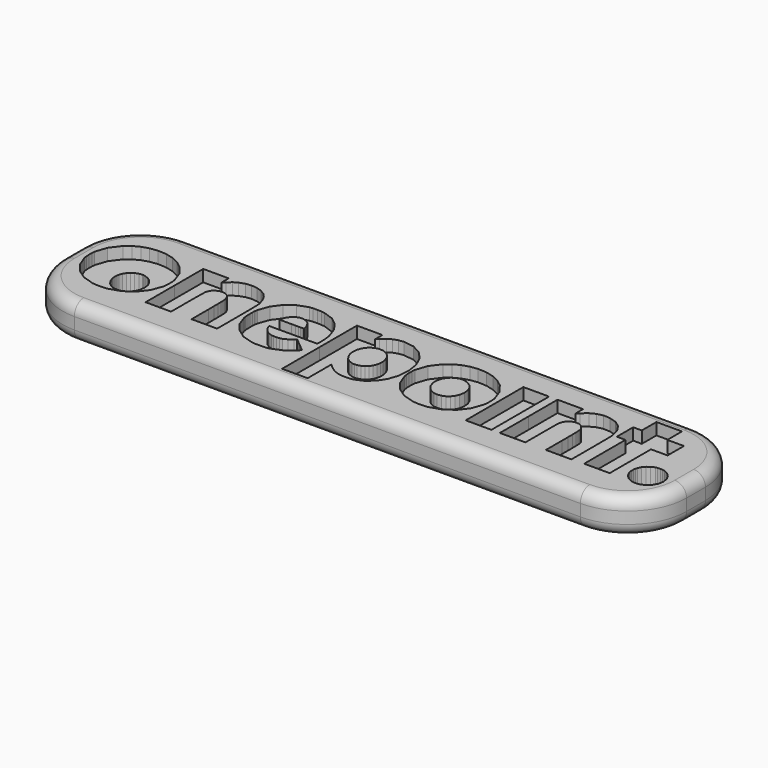
from build123d import *

# Parameters (mm, degrees)
F0_W     = 52.8722088784
F0_H     = 12
F1_DEPTH = 3
F2_DEPTH = 1
F3_R     = 5
F4_DEPTH = 3
F5_R     = 1
F6_R     = 1


# Not quite as in the source:
# - a feature names something its author has since deleted; it is built from what else it names


with BuildPart() as f1:
    # F0 (on Top) → F1 (new body)
    with BuildSketch(Plane.XY):
        with Locations((0.0200578943, 0)):
            Rectangle(F0_W, F0_H)
        Polygon((-4.8085591433, -0.7883964354), (-4.8082865964, -0.7883964354), (-4.8082865964, 3.167022304), (-2.6444276898, 3.167022304), (-2.6444276898, 2.3789256702), (-2.4436151294, 2.5936381229), (-2.0997154432, 2.8928946258), (-1.743660165, 3.1061898346), (-1.3576792365, 3.2388656685), (-0.9247112214, 3.2959369906), (-0.0383886827, 3.1815763088), (0.7376068685, 2.7766806251), (1.3524181794, 2.1192429781), (1.7551879973, 1.2465477846), (1.9036170423, 0.2741549329), (1.8268133242, -0.730998057), (1.5597173562, -1.5324494892), (1.1208078185, -2.1981180527), (0.5367943081, -2.6997133788), (-0.1652865222, -3.0096537204), (-0.3063568008, -3.0427409148), (-0.4323279808, -3.0595843136), (-0.5826103448, -3.0657983831), (-0.7957965348, -3.0669430801), (-1.017595207, -3.0657983831), (-1.170439512, -3.0595843136), (-1.2937942417, -3.0427409148), (-1.4262520381, -3.0096537204), (-1.7128078552, -2.9111552686), (-1.9763607135, -2.7819135257), (-2.2265042639, -2.6124983688), (-2.4725596108, -2.3933161469), (-2.6444276898, -2.2356750164), (-2.6444276898, -4.7579331046), (-4.8085591433, -4.7579331046), align=None, mode=Mode.SUBTRACT)
        Polygon((23.3377414195, -2.9093019496), (23.3371963256, -2.9093019496), (23.0014730467, -2.7620721109), (22.7173156423, -2.5293715624), (22.5026031897, -2.2318048503), (22.3769045565, -1.8917208208), (22.3636042675, -1.7213790045), (22.3680740368, -1.5297785295), (22.391131505, -1.3434654644), (22.4352295945, -1.1894219531), (22.5715030475, -0.9104974493), (22.7643027289, -0.6771427883), (23.010957679, -0.492083439), (23.3091239943, -0.3583719269), (23.4737423256, -0.3258298263), (23.6813685587, -0.315200497), (23.8893218481, -0.3258298263), (24.0542672357, -0.3583719269), (24.4497327965, -0.5594570342), (24.7475175462, -0.8507551675), (24.9347027613, -1.2148233247), (25.000005, -1.6338914476), (24.9261447884, -2.0606453933), (24.722334212, -2.4379593301), (24.4135930767, -2.7319284231), (24.0255953012, -2.9093019496), (23.8674635862, -2.9333405867), (23.6757540924, -2.9412989564), (23.487097124, -2.9333405867), align=None, mode=Mode.SUBTRACT)
        Polygon((-22.2201146743, -3.0240987065), (-22.2201146743, -3.0237716502), (-23.191886119, -2.7287123696), (-23.9953925549, -2.1889604767), (-24.5921830643, -1.4398380504), (-24.9429182269, -0.515958548), (-24.9837294006, -0.2705573137), (-24.999995, 0.0270093984), (-24.9952635857, 0.3327525177), (-24.9713067127, 0.6018108234), (-24.6489600358, 1.5727864313), (-24.0252582449, 2.3931526187), (-23.5512010582, 2.774663778), (-23.0150413335, 3.0576219759), (-22.4253479455, 3.2415911376), (-21.7898230698, 3.3246634346), (-21.0584761528, 3.2880331304), (-20.3765147352, 3.1170917108), (-19.7563669559, 2.8169085484), (-19.2101502503, 2.3931526187), (-18.6118825367, 1.6049469662), (-18.2930844206, 0.6879356458), (-18.2635130813, 0.4265086534), (-18.2575933625, 0.1219102311), (-18.2732702605, -0.1827427006), (-18.3078673648, -0.4444422398), (-18.6444137354, -1.3751354149), (-19.2358786783, -2.1404471274), (-20.0370139561, -2.6990592662), (-21.001993532, -3.0096537204), (-21.6168157447, -3.0542423943), align=None, mode=Mode.SUBTRACT)
        Polygon((-17.8210931395, 0.1002700068), (-17.8205044381, 0.1002700068), (-17.8205044381, 3.152577318), (-15.6566346297, 3.152577318), (-15.6566346297, 2.3644806842), (-15.4274226816, 2.5936381229), (-15.1086518202, 2.8857538969), (-14.7682407344, 3.0810065005), (-14.3237712399, 3.2424632877), (-13.8331322994, 3.2977903096), (-13.3374784959, 3.2484048102), (-12.8764381495, 3.0951789396), (-12.4913838805, 2.8550651153), (-12.1906556243, 2.5365122914), (-11.9676577457, 2.1322707202), (-11.8159036283, 1.6336734101), (-11.8017311892, 1.5656457023), (-11.7907748036, 1.467801363), (-11.7828164339, 1.3219887682), (-11.7766023645, 1.1104923691), (-11.7718600483, 0.8162507292), (-11.7680443916, 0.4205671309), (-11.7642287349, -0.0940014279), (-11.7594319094, -0.7451704961), (-11.7594319094, -2.952255342), (-13.9233453254, -2.952255342), (-13.9233453254, -1.1751950046), (-13.9283601884, -0.5916720785), (-13.9327754483, -0.1492739405), (-13.9369181613, 0.1739121808), (-13.9416604775, 0.3996355285), (-13.9482016032, 0.5492092706), (-13.9561599729, 0.6447642159), (-13.9671163585, 0.7077770606), (-13.9812887976, 0.759451954), (-14.0975027984, 1.0067065072), (-14.2539447225, 1.1894764625), (-14.4530129828, 1.3078163291), (-14.6978691232, 1.3613445415), (-14.9862237499, 1.3444466333), (-15.2408370696, 1.2358639459), (-15.4496079997, 1.0472069775), (-15.6007625139, 0.7881238885), (-15.6152074999, 0.7408097456), (-15.6261638855, 0.68139452), (-15.6341767646, 0.5879654406), (-15.6403363247, 0.4389367923), (-15.6450786408, 0.2127228602), (-15.6489488069, -0.1125891269), (-15.6527644636, -0.5583123372), (-15.6572342328, -1.1464685607), (-15.6572342328, -2.952255342), (-17.8210931395, -2.952255342), align=None, mode=Mode.SUBTRACT)
        Polygon((-8.6758907227, -3.0524980941), (-8.6776350229, -3.0524980941), (-9.6970149612, -2.7478996718), (-10.5120937387, -2.1641587082), (-11.0334759702, -1.472380151), (-11.3285897601, -0.6307553049), (-11.3557899414, -0.4902301201), (-11.3732329434, -0.3474700506), (-11.3827175757, -0.1670439988), (-11.3853885354, 0.0858250207), (-11.3823905194, 0.3451806566), (-11.3726333402, 0.5250071053), (-11.3552448476, 0.6646056306), (-11.3285897601, 0.8024053464), (-11.0118357458, 1.6928705981), (-10.4689223088, 2.4218245533), (-9.7632438594, 2.9555804143), (-8.9068469709, 3.253092617), (-8.6205091914, 3.2850351144), (-8.2600931627, 3.2942471998), (-7.8972242118, 3.2791481012), (-7.6026555157, 3.238647631), (-6.7645737793, 2.9502930043), (-6.0979785563, 2.4363240487), (-5.6126815352, 1.7324444089), (-5.3098274131, 0.8455222669), (-5.2702536023, 0.5696502885), (-5.2400554051, 0.2384512882), (-5.2234845532, -0.0792293856), (-5.2234845532, -0.315200497), (-5.2518294315, -0.501513562), (-9.3075999417, -0.501513562), (-9.2924463338, -0.5589119404), (-9.2655732088, -0.6446006877), (-9.2061034739, -0.7738424306), (-9.0623622356, -1.0037084912), (-8.8713613638, -1.1947093631), (-8.6400780592, -1.3399223547), (-8.3751079571, -1.4330243778), (-8.1636115579, -1.4606061247), (-7.9184828705, -1.4600065215), (-7.6760251428, -1.4351502437), (-7.4722690758, -1.3901800041), (-7.1499005952, -1.2269789168), (-6.8272595677, -0.9888819395), (-6.6553914887, -0.8454677575), (-6.0532808637, -1.3470085742), (-5.4514972949, -1.8486039003), (-5.5662395424, -1.9778456432), (-6.3348218177, -2.6278700143), (-7.2859560107, -3.0096537204), (-7.4329133025, -3.0365268454), (-7.5798705943, -3.0540243568), (-7.7697267691, -3.063781536), (-8.04538071, -3.0667250426), (-8.2488097208, -3.0723395088), (-8.4360494453, -3.070213643), (-8.5857322061, -3.0625823296), align=None, mode=Mode.SUBTRACT)
        Polygon((5.5113204389, -3.0542423943), (4.9080106075, -3.0237716502), (3.936217359, -2.7287123696), (3.1327490797, -2.1889604767), (2.5359258646, -1.4398380504), (2.1852125058, -0.515958548), (2.1443849792, -0.2705573137), (2.1278141273, 0.0270093984), (2.1328834998, 0.3327525177), (2.1568131181, 0.6018108234), (2.4791815987, 1.5727864313), (3.1028234294, 2.3931526187), (3.5769460273, 2.774663778), (4.113100301, 3.0576219759), (4.7027827872, 3.2415911376), (5.3382531535, 3.3246634346), (6.0696600308, 3.2880331304), (6.75157239, 3.1170917108), (7.3714530733, 2.8169085484), (7.9176915826, 2.3931526187), (8.5159320416, 1.6049469662), (8.8350299593, 0.6879356458), (8.8646285533, 0.4265086534), (8.8705700759, 0.1219102311), (8.8548713741, -0.1827427006), (8.820257917, -0.4444422398), (8.4836624879, -1.3751354149), (7.8919631547, -2.1404471274), (7.0908387788, -2.6990592662), (6.1258592029, -3.0096537204), align=None, mode=Mode.SUBTRACT)
        Polygon((9.2931267991, -2.9377013372), (9.2931267991, 0.1144969553), (9.2931267991, 3.167022304), (11.4714852012, 3.167022304), (11.4714852012, -2.9377013372), align=None, mode=Mode.SUBTRACT)
        Polygon((12.186811811, 0.1144969553), (12.1880655268, 0.1144969553), (12.1880655268, 3.167022304), (14.3519244334, 3.167022304), (14.3519244334, 2.3501992263), (14.5810818721, 2.5794656838), (15.0143769435, 2.9532365109), (15.4801050967, 3.1940044477), (15.9837717792, 3.3030777196), (16.530228326, 3.2814920046), (17.1752923435, 3.08809272), (17.6818480232, 2.7119779895), (18.0352323417, 2.16928259), (18.221000313, 1.4760322796), (18.2316296423, 1.248891688), (18.2404601621, 0.754164544), (18.2470012878, 0.0473413976), (18.2493451912, -0.8170683699), (18.2493451912, -2.9377013372), (16.0852137377, -2.9377013372), (16.0852137377, -1.2038669391), (16.0849411908, -0.5769545456), (16.0831423812, -0.0996158942), (16.0781275181, 0.2516970678), (16.0689699421, 0.5016225808), (16.0535982966, 0.6734361504), (16.0304863189, 0.7913944514), (15.9982712746, 0.878991027), (15.9556994479, 0.9599919675), (15.7593021473, 1.2034308641), (15.4917155949, 1.347117593), (15.1837921003, 1.3835298596), (14.8668200485, 1.303946163), (14.6334653874, 1.1356757032), (14.4651949276, 0.9026480984), (14.4273109076, 0.8157056354), (14.39891152, 0.7224945935), (14.3785795208, 0.6000665232), (14.3649521755, 0.4265086534), (14.3566667496, 0.1787090064), (14.3525240366, -0.1652451892), (14.350725227, -0.6280843452), (14.350725227, -1.2325388736), (14.350725227, -2.9377013372), (12.186811811, -2.9377013372), align=None, mode=Mode.SUBTRACT)
        Polygon((19.2957072732, -2.8948569636), (19.2957072732, -0.7165530709), (19.2957072732, 1.4760322796), (18.5648999991, 1.4760322796), (18.5648999991, 3.2099756964), (19.2957072732, 3.2099756964), (19.2957072732, 4.7579331046), (21.4595661799, 4.7579331046), (21.4595661799, 3.2099756964), (22.8643274435, 3.2099756964), (22.8643274435, 1.4760322796), (21.4595661799, 1.4760322796), (21.4595661799, -2.8948569636), align=None, mode=Mode.SUBTRACT)
        Polygon((-4.8082865964, 3.167022304), (-4.8082865964, -0.7883964354), (-4.8085591433, -0.7883964354), (-4.8085591433, -4.7579331046), (-2.6444276898, -4.7579331046), (-2.6444276898, -2.2356750164), (-2.4725596108, -2.3933161469), (-2.2265042639, -2.6124983688), (-1.9763607135, -2.7819135257), (-1.7128078552, -2.9111552686), (-1.4262520381, -3.0096537204), (-1.2937942417, -3.0427409148), (-1.170439512, -3.0595843136), (-1.017595207, -3.0657983831), (-0.7957965348, -3.0669430801), (-0.5826103448, -3.0657983831), (-0.4323279808, -3.0595843136), (-0.3063568008, -3.0427409148), (-0.1652865222, -3.0096537204), (0.5367943081, -2.6997133788), (1.1208078185, -2.1981180527), (1.5597173562, -1.5324494892), (1.8268133242, -0.730998057), (1.9036170423, 0.2741549329), (1.7551879973, 1.2465477846), (1.3524181794, 2.1192429781), (0.7376068685, 2.7766806251), (-0.0383886827, 3.1815763088), (-0.9247112214, 3.2959369906), (-1.3576792365, 3.2388656685), (-1.743660165, 3.1061898346), (-2.0997154432, 2.8928946258), (-2.4436151294, 2.5936381229), (-2.6444276898, 2.3789256702), (-2.6444276898, 3.167022304), align=None)
        Polygon((-1.0051670681, -1.1766667579), (-1.2541659216, -1.2467658221), (-1.481851607, -1.2680789902), (-1.6986899255, -1.2467658221), (-2.0156619773, -1.1225389423), (-2.2880453553, -0.9098978461), (-2.498615095, -0.6219247851), (-2.6299281944, -0.2723016139), (-2.6618161824, -0.0986892347), (-2.6725000211, 0.1148240116), (-2.6618161824, 0.3282827484), (-2.6299281944, 0.5016225808), (-2.4852602966, 0.8614935156), (-2.2576291206, 1.1554626086), (-1.9650772716, 1.3660323483), (-1.626846561, 1.4760322796), (-1.1787794473, 1.4530293207), (-0.7815695863, 1.2702593654), (-0.4701574914, 0.9502347883), (-0.2797562227, 0.5158495293), (-0.2312428735, 0.2260231493), (-0.2351130395, -0.0733423724), (-0.2900584958, -0.3648585432), (-0.3944439608, -0.6307553049), (-0.5553556542, -0.8536986741), (-0.7653257907, -1.0406658517), align=None, mode=Mode.SUBTRACT)
        Polygon((-23.191886119, -2.7287123696), (-22.2201146743, -3.0237716502), (-22.2201146743, -3.0240987065), (-21.6168157447, -3.0542423943), (-21.001993532, -3.0096537204), (-20.0370139561, -2.6990592662), (-19.2358786783, -2.1404471274), (-18.6444137354, -1.3751354149), (-18.3078673648, -0.4444422398), (-18.2732702605, -0.1827427006), (-18.2575933625, 0.1219102311), (-18.2635130813, 0.4265086534), (-18.2930844206, 0.6879356458), (-18.6118825367, 1.6049469662), (-19.2101502503, 2.3931526187), (-19.7563669559, 2.8169085484), (-20.3765147352, 3.1170917108), (-21.0584761528, 3.2880331304), (-21.7898230698, 3.3246634346), (-22.4253479455, 3.2415911376), (-23.0150413335, 3.0576219759), (-23.5512010582, 2.774663778), (-24.0252582449, 2.3931526187), (-24.6489600358, 1.5727864313), (-24.9713067127, 0.6018108234), (-24.9952635857, 0.3327525177), (-24.999995, 0.0270093984), (-24.9837294006, -0.2705573137), (-24.9429182269, -0.515958548), (-24.5921830643, -1.4398380504), (-23.9953925549, -2.1889604767), align=None)
        Polygon((-21.0155936226, -1.0734259898), (-21.3030488445, -1.1894219531), (-21.3033431951, -1.1894219531), (-21.6239183171, -1.221582488), (-21.9338423059, -1.1894219531), (-22.24850316, -1.0551108377), (-22.5161387709, -0.8365827284), (-22.7216772947, -0.5505720051), (-22.8509081357, -0.2149577449), (-22.8837336851, -0.0564444643), (-22.8943793672, 0.1399528363), (-22.8837336851, 0.3413104906), (-22.8509081357, 0.5158495293), (-22.7624830175, 0.7710624522), (-22.614615419, 1.0085598262), (-22.4238707413, 1.2110621774), (-22.2059204314, 1.3613445415), (-21.9214250689, 1.4600610309), (-21.6472810379, 1.5047042141), (-21.5417018174, 1.4941293942), (-21.4035968491, 1.4615872936), (-21.0717818927, 1.3424297862), (-20.7911348925, 1.1410176226), (-20.5693362203, 0.8674350382), (-20.4146658511, 0.5302945153), (-20.364986001, 0.091439487), (-20.4430543368, -0.3583719269), (-20.5855963688, -0.6594272394), (-20.7763464974, -0.8974697072), align=None, mode=Mode.SUBTRACT)
        Polygon((3.936217359, -2.7287123696), (4.9080106075, -3.0237716502), (5.5113204389, -3.0542423943), (6.1258592029, -3.0096537204), (7.0908387788, -2.6990592662), (7.8919631547, -2.1404471274), (8.4836624879, -1.3751354149), (8.820257917, -0.4444422398), (8.8548713741, -0.1827427006), (8.8705700759, 0.1219102311), (8.8646285533, 0.4265086534), (8.8350299593, 0.6879356458), (8.5159320416, 1.6049469662), (7.9176915826, 2.3931526187), (7.3714530733, 2.8169085484), (6.75157239, 3.1170917108), (6.0696600308, 3.2880331304), (5.3382531535, 3.3246634346), (4.7027827872, 3.2415911376), (4.113100301, 3.0576219759), (3.5769460273, 2.774663778), (3.1028234294, 2.3931526187), (2.4791815987, 1.5727864313), (2.1568131181, 0.6018108234), (2.1328834998, 0.3327525177), (2.1278141273, 0.0270093984), (2.1443849792, -0.2705573137), (2.1852125058, -0.515958548), (2.5359258646, -1.4398380504), (3.1327490797, -2.1889604767), align=None)
        Polygon((6.1125044045, -1.0734259898), (5.8250764373, -1.1894219531), (5.824749381, -1.1894219531), (5.5042342194, -1.221582488), (5.1942938777, -1.1894219531), (4.8796112199, -1.0551108377), (4.6120246674, -0.8365827284), (4.4061427345, -0.5505720051), (4.2772280479, -0.2149577449), (4.244358891, -0.0564444643), (4.2337840711, 0.1399528363), (4.244358891, 0.3413104906), (4.2772280479, 0.5158495293), (4.3656422643, 0.7710624522), (4.5135262155, 1.0085598262), (4.7042000311, 1.2110621774), (4.9218559903, 1.3613445415), (5.2066675072, 1.4600610309), (5.4807951854, 1.5047042141), (5.58610731, 1.4941293942), (5.7245066289, 1.4615872936), (6.0560326855, 1.3424297862), (6.3369740364, 1.1410176226), (6.5585001617, 0.8674350382), (6.7131977856, 0.5302945153), (6.7631283788, 0.091439487), (6.6850164355, -0.3583719269), (6.542528913, -0.6594272394), (6.3517460787, -0.8974697072), align=None, mode=Mode.SUBTRACT)
        Polygon((-17.8205044381, 3.152577318), (-17.8205044381, 0.1002700068), (-17.8210931395, 0.1002700068), (-17.8210931395, -2.952255342), (-15.6572342328, -2.952255342), (-15.6572342328, -1.1464685607), (-15.6527644636, -0.5583123372), (-15.6489488069, -0.1125891269), (-15.6450786408, 0.2127228602), (-15.6403363247, 0.4389367923), (-15.6341767646, 0.5879654406), (-15.6261638855, 0.68139452), (-15.6152074999, 0.7408097456), (-15.6007625139, 0.7881238885), (-15.4496079997, 1.0472069775), (-15.2408370696, 1.2358639459), (-14.9862237499, 1.3444466333), (-14.6978691232, 1.3613445415), (-14.4530129828, 1.3078163291), (-14.2539447225, 1.1894764625), (-14.0975027984, 1.0067065072), (-13.9812887976, 0.759451954), (-13.9671163585, 0.7077770606), (-13.9561599729, 0.6447642159), (-13.9482016032, 0.5492092706), (-13.9416604775, 0.3996355285), (-13.9369181613, 0.1739121808), (-13.9327754483, -0.1492739405), (-13.9283601884, -0.5916720785), (-13.9233453254, -1.1751950046), (-13.9233453254, -2.952255342), (-11.7594319094, -2.952255342), (-11.7594319094, -0.7451704961), (-11.7642287349, -0.0940014279), (-11.7680443916, 0.4205671309), (-11.7718600483, 0.8162507292), (-11.7766023645, 1.1104923691), (-11.7828164339, 1.3219887682), (-11.7907748036, 1.467801363), (-11.8017311892, 1.5656457023), (-11.8159036283, 1.6336734101), (-11.9676577457, 2.1322707202), (-12.1906556243, 2.5365122914), (-12.4913838805, 2.8550651153), (-12.8764381495, 3.0951789396), (-13.3374784959, 3.2484048102), (-13.8331322994, 3.2977903096), (-14.3237712399, 3.2424632877), (-14.7682407344, 3.0810065005), (-15.1086518202, 2.8857538969), (-15.4274226816, 2.5936381229), (-15.6566346297, 2.3644806842), (-15.6566346297, 3.152577318), align=None)
        Polygon((12.1880655268, 3.167022304), (12.1880655268, 0.1144969553), (12.186811811, 0.1144969553), (12.186811811, -2.9377013372), (14.350725227, -2.9377013372), (14.350725227, -1.2325388736), (14.350725227, -0.6280843452), (14.3525240366, -0.1652451892), (14.3566667496, 0.1787090064), (14.3649521755, 0.4265086534), (14.3785795208, 0.6000665232), (14.39891152, 0.7224945935), (14.4273109076, 0.8157056354), (14.4651949276, 0.9026480984), (14.6334653874, 1.1356757032), (14.8668200485, 1.303946163), (15.1837921003, 1.3835298596), (15.4917155949, 1.347117593), (15.7593021473, 1.2034308641), (15.9556994479, 0.9599919675), (15.9982712746, 0.878991027), (16.0304863189, 0.7913944514), (16.0535982966, 0.6734361504), (16.0689699421, 0.5016225808), (16.0781275181, 0.2516970678), (16.0831423812, -0.0996158942), (16.0849411908, -0.5769545456), (16.0852137377, -1.2038669391), (16.0852137377, -2.9377013372), (18.2493451912, -2.9377013372), (18.2493451912, -0.8170683699), (18.2470012878, 0.0473413976), (18.2404601621, 0.754164544), (18.2316296423, 1.248891688), (18.221000313, 1.4760322796), (18.0352323417, 2.16928259), (17.6818480232, 2.7119779895), (17.1752923435, 3.08809272), (16.530228326, 3.2814920046), (15.9837717792, 3.3030777196), (15.4801050967, 3.1940044477), (15.0143769435, 2.9532365109), (14.5810818721, 2.5794656838), (14.3519244334, 2.3501992263), (14.3519244334, 3.167022304), align=None)
        Polygon((-9.6970149612, -2.7478996718), (-8.6776350229, -3.0524980941), (-8.6758907227, -3.0524980941), (-8.5857322061, -3.0625823296), (-8.4360494453, -3.070213643), (-8.2488097208, -3.0723395088), (-8.04538071, -3.0667250426), (-7.7697267691, -3.063781536), (-7.5798705943, -3.0540243568), (-7.4329133025, -3.0365268454), (-7.2859560107, -3.0096537204), (-6.3348218177, -2.6278700143), (-5.5662395424, -1.9778456432), (-5.4514972949, -1.8486039003), (-6.0532808637, -1.3470085742), (-6.6553914887, -0.8454677575), (-6.8272595677, -0.9888819395), (-7.1499005952, -1.2269789168), (-7.4722690758, -1.3901800041), (-7.6760251428, -1.4351502437), (-7.9184828705, -1.4600065215), (-8.1636115579, -1.4606061247), (-8.3751079571, -1.4330243778), (-8.6400780592, -1.3399223547), (-8.8713613638, -1.1947093631), (-9.0623622356, -1.0037084912), (-9.2061034739, -0.7738424306), (-9.2655732088, -0.6446006877), (-9.2924463338, -0.5589119404), (-9.3075999417, -0.501513562), (-5.2518294315, -0.501513562), (-5.2234845532, -0.315200497), (-5.2234845532, -0.0792293856), (-5.2400554051, 0.2384512882), (-5.2702536023, 0.5696502885), (-5.3098274131, 0.8455222669), (-5.6126815352, 1.7324444089), (-6.0979785563, 2.4363240487), (-6.7645737793, 2.9502930043), (-7.6026555157, 3.238647631), (-7.8972242118, 3.2791481012), (-8.2600931627, 3.2942471998), (-8.6205091914, 3.2850351144), (-8.9068469709, 3.253092617), (-9.7632438594, 2.9555804143), (-10.4689223088, 2.4218245533), (-11.0118357458, 1.6928705981), (-11.3285897601, 0.8024053464), (-11.3552448476, 0.6646056306), (-11.3726333402, 0.5250071053), (-11.3823905194, 0.3451806566), (-11.3853885354, 0.0858250207), (-11.3827175757, -0.1670439988), (-11.3732329434, -0.3474700506), (-11.3557899414, -0.4902301201), (-11.3285897601, -0.6307553049), (-11.0334759702, -1.472380151), (-10.5120937387, -2.1641587082), align=None)
        Polygon((-7.2734733624, 0.7514935843), (-7.2587013201, 0.6592092019), (-7.2590283764, 0.6592092019), (-7.2652424459, 0.6497790789), (-7.2894446111, 0.6426928594), (-7.3406289201, 0.6376234869), (-7.4276258926, 0.6344074334), (-7.5585574263, 0.6323360769), (-7.7428536442, 0.6311368705), (-7.9885819348, 0.6308098143), (-8.3050634022, 0.6305372674), (-9.3513164655, 0.6305372674), (-9.3081995449, 0.8024053464), (-9.1741609765, 1.1410176226), (-8.9875753645, 1.4027716712), (-8.7500779905, 1.5866318141), (-8.4627045327, 1.6910172791), (-8.1440971994, 1.6928705981), (-7.8481112594, 1.5961164464), (-7.5982402558, 1.4110025878), (-7.4163424506, 1.1463050325), (-7.3618875788, 1.0220781527), (-7.3110848355, 0.8813349304), align=None, mode=Mode.SUBTRACT)
        Polygon((19.2957072732, 1.4760322796), (19.2957072732, -0.7165530709), (19.2957072732, -2.8948569636), (21.4595661799, -2.8948569636), (21.4595661799, 1.4760322796), (22.8643274435, 1.4760322796), (22.8643274435, 3.2099756964), (21.4595661799, 3.2099756964), (21.4595661799, 4.7579331046), (19.2957072732, 4.7579331046), (19.2957072732, 3.2099756964), (18.5648999991, 3.2099756964), (18.5648999991, 1.4760322796), align=None)
        Polygon((9.2931267991, 3.167022304), (9.2931267991, 0.1144969553), (9.2931267991, -2.9377013372), (11.4714852012, -2.9377013372), (11.4714852012, 3.167022304), align=None)
        Polygon((23.0014730467, -2.7620721109), (23.3371963256, -2.9093019496), (23.3377414195, -2.9093019496), (23.487097124, -2.9333405867), (23.6757540924, -2.9412989564), (23.8674635862, -2.9333405867), (24.0255953012, -2.9093019496), (24.4135930767, -2.7319284231), (24.722334212, -2.4379593301), (24.9261447884, -2.0606453933), (25.000005, -1.6338914476), (24.9347027613, -1.2148233247), (24.7475175462, -0.8507551675), (24.4497327965, -0.5594570342), (24.0542672357, -0.3583719269), (23.8893218481, -0.3258298263), (23.6813685587, -0.315200497), (23.4737423256, -0.3258298263), (23.3091239943, -0.3583719269), (23.010957679, -0.492083439), (22.7643027289, -0.6771427883), (22.5715030475, -0.9104974493), (22.4352295945, -1.1894219531), (22.391131505, -1.3434654644), (22.3680740368, -1.5297785295), (22.3636042675, -1.7213790045), (22.3769045565, -1.8917208208), (22.5026031897, -2.2318048503), (22.7173156423, -2.5293715624), align=None)
        Polygon((5.824749381, -1.1894219531), (5.8250764373, -1.1894219531), (6.1125044045, -1.0734259898), (6.3517460787, -0.8974697072), (6.542528913, -0.6594272394), (6.6850164355, -0.3583719269), (6.7631283788, 0.091439487), (6.7131977856, 0.5302945153), (6.5585001617, 0.8674350382), (6.3369740364, 1.1410176226), (6.0560326855, 1.3424297862), (5.7245066289, 1.4615872936), (5.58610731, 1.4941293942), (5.4807951854, 1.5047042141), (5.2066675072, 1.4600610309), (4.9218559903, 1.3613445415), (4.7042000311, 1.2110621774), (4.5135262155, 1.0085598262), (4.3656422643, 0.7710624522), (4.2772280479, 0.5158495293), (4.244358891, 0.3413104906), (4.2337840711, 0.1399528363), (4.244358891, -0.0564444643), (4.2772280479, -0.2149577449), (4.4061427345, -0.5505720051), (4.6120246674, -0.8365827284), (4.8796112199, -1.0551108377), (5.1942938777, -1.1894219531), (5.5042342194, -1.221582488), align=None)
        Polygon((-1.481851607, -1.2680789902), (-1.2541659216, -1.2467658221), (-1.0051670681, -1.1766667579), (-0.7653257907, -1.0406658517), (-0.5553556542, -0.8536986741), (-0.3944439608, -0.6307553049), (-0.2900584958, -0.3648585432), (-0.2351130395, -0.0733423724), (-0.2312428735, 0.2260231493), (-0.2797562227, 0.5158495293), (-0.4701574914, 0.9502347883), (-0.7815695863, 1.2702593654), (-1.1787794473, 1.4530293207), (-1.626846561, 1.4760322796), (-1.9650772716, 1.3660323483), (-2.2576291206, 1.1554626086), (-2.4852602966, 0.8614935156), (-2.6299281944, 0.5016225808), (-2.6618161824, 0.3282827484), (-2.6725000211, 0.1148240116), (-2.6618161824, -0.0986892347), (-2.6299281944, -0.2723016139), (-2.498615095, -0.6219247851), (-2.2880453553, -0.9098978461), (-2.0156619773, -1.1225389423), (-1.6986899255, -1.2467658221), align=None)
        Polygon((-7.2590283764, 0.6592092019), (-7.2587013201, 0.6592092019), (-7.2734733624, 0.7514935843), (-7.3110848355, 0.8813349304), (-7.3618875788, 1.0220781527), (-7.4163424506, 1.1463050325), (-7.5982402558, 1.4110025878), (-7.8481112594, 1.5961164464), (-8.1440971994, 1.6928705981), (-8.4627045327, 1.6910172791), (-8.7500779905, 1.5866318141), (-8.9875753645, 1.4027716712), (-9.1741609765, 1.1410176226), (-9.3081995449, 0.8024053464), (-9.3513164655, 0.6305372674), (-8.3050634022, 0.6305372674), (-7.9885819348, 0.6308098143), (-7.7428536442, 0.6311368705), (-7.5585574263, 0.6323360769), (-7.4276258926, 0.6344074334), (-7.3406289201, 0.6376234869), (-7.2894446111, 0.6426928594), (-7.2652424459, 0.6497790789), align=None)
    extrude(amount=-F1_DEPTH)

    # F0 (on Top) → F2 (cut)
    with BuildSketch(Plane.XY):
        Polygon((-23.191886119, -2.7287123696), (-22.2201146743, -3.0237716502), (-22.2201146743, -3.0240987065), (-21.6168157447, -3.0542423943), (-21.001993532, -3.0096537204), (-20.0370139561, -2.6990592662), (-19.2358786783, -2.1404471274), (-18.6444137354, -1.3751354149), (-18.3078673648, -0.4444422398), (-18.2732702605, -0.1827427006), (-18.2575933625, 0.1219102311), (-18.2635130813, 0.4265086534), (-18.2930844206, 0.6879356458), (-18.6118825367, 1.6049469662), (-19.2101502503, 2.3931526187), (-19.7563669559, 2.8169085484), (-20.3765147352, 3.1170917108), (-21.0584761528, 3.2880331304), (-21.7898230698, 3.3246634346), (-22.4253479455, 3.2415911376), (-23.0150413335, 3.0576219759), (-23.5512010582, 2.774663778), (-24.0252582449, 2.3931526187), (-24.6489600358, 1.5727864313), (-24.9713067127, 0.6018108234), (-24.9952635857, 0.3327525177), (-24.999995, 0.0270093984), (-24.9837294006, -0.2705573137), (-24.9429182269, -0.515958548), (-24.5921830643, -1.4398380504), (-23.9953925549, -2.1889604767), align=None)
        Polygon((-21.0155936226, -1.0734259898), (-21.3030488445, -1.1894219531), (-21.3033431951, -1.1894219531), (-21.6239183171, -1.221582488), (-21.9338423059, -1.1894219531), (-22.24850316, -1.0551108377), (-22.5161387709, -0.8365827284), (-22.7216772947, -0.5505720051), (-22.8509081357, -0.2149577449), (-22.8837336851, -0.0564444643), (-22.8943793672, 0.1399528363), (-22.8837336851, 0.3413104906), (-22.8509081357, 0.5158495293), (-22.7624830175, 0.7710624522), (-22.614615419, 1.0085598262), (-22.4238707413, 1.2110621774), (-22.2059204314, 1.3613445415), (-21.9214250689, 1.4600610309), (-21.6472810379, 1.5047042141), (-21.5417018174, 1.4941293942), (-21.4035968491, 1.4615872936), (-21.0717818927, 1.3424297862), (-20.7911348925, 1.1410176226), (-20.5693362203, 0.8674350382), (-20.4146658511, 0.5302945153), (-20.364986001, 0.091439487), (-20.4430543368, -0.3583719269), (-20.5855963688, -0.6594272394), (-20.7763464974, -0.8974697072), align=None, mode=Mode.SUBTRACT)
        Polygon((-17.8205044381, 3.152577318), (-17.8205044381, 0.1002700068), (-17.8210931395, 0.1002700068), (-17.8210931395, -2.952255342), (-15.6572342328, -2.952255342), (-15.6572342328, -1.1464685607), (-15.6527644636, -0.5583123372), (-15.6489488069, -0.1125891269), (-15.6450786408, 0.2127228602), (-15.6403363247, 0.4389367923), (-15.6341767646, 0.5879654406), (-15.6261638855, 0.68139452), (-15.6152074999, 0.7408097456), (-15.6007625139, 0.7881238885), (-15.4496079997, 1.0472069775), (-15.2408370696, 1.2358639459), (-14.9862237499, 1.3444466333), (-14.6978691232, 1.3613445415), (-14.4530129828, 1.3078163291), (-14.2539447225, 1.1894764625), (-14.0975027984, 1.0067065072), (-13.9812887976, 0.759451954), (-13.9671163585, 0.7077770606), (-13.9561599729, 0.6447642159), (-13.9482016032, 0.5492092706), (-13.9416604775, 0.3996355285), (-13.9369181613, 0.1739121808), (-13.9327754483, -0.1492739405), (-13.9283601884, -0.5916720785), (-13.9233453254, -1.1751950046), (-13.9233453254, -2.952255342), (-11.7594319094, -2.952255342), (-11.7594319094, -0.7451704961), (-11.7642287349, -0.0940014279), (-11.7680443916, 0.4205671309), (-11.7718600483, 0.8162507292), (-11.7766023645, 1.1104923691), (-11.7828164339, 1.3219887682), (-11.7907748036, 1.467801363), (-11.8017311892, 1.5656457023), (-11.8159036283, 1.6336734101), (-11.9676577457, 2.1322707202), (-12.1906556243, 2.5365122914), (-12.4913838805, 2.8550651153), (-12.8764381495, 3.0951789396), (-13.3374784959, 3.2484048102), (-13.8331322994, 3.2977903096), (-14.3237712399, 3.2424632877), (-14.7682407344, 3.0810065005), (-15.1086518202, 2.8857538969), (-15.4274226816, 2.5936381229), (-15.6566346297, 2.3644806842), (-15.6566346297, 3.152577318), align=None)
        Polygon((-9.6970149612, -2.7478996718), (-8.6776350229, -3.0524980941), (-8.6758907227, -3.0524980941), (-8.5857322061, -3.0625823296), (-8.4360494453, -3.070213643), (-8.2488097208, -3.0723395088), (-8.04538071, -3.0667250426), (-7.7697267691, -3.063781536), (-7.5798705943, -3.0540243568), (-7.4329133025, -3.0365268454), (-7.2859560107, -3.0096537204), (-6.3348218177, -2.6278700143), (-5.5662395424, -1.9778456432), (-5.4514972949, -1.8486039003), (-6.0532808637, -1.3470085742), (-6.6553914887, -0.8454677575), (-6.8272595677, -0.9888819395), (-7.1499005952, -1.2269789168), (-7.4722690758, -1.3901800041), (-7.6760251428, -1.4351502437), (-7.9184828705, -1.4600065215), (-8.1636115579, -1.4606061247), (-8.3751079571, -1.4330243778), (-8.6400780592, -1.3399223547), (-8.8713613638, -1.1947093631), (-9.0623622356, -1.0037084912), (-9.2061034739, -0.7738424306), (-9.2655732088, -0.6446006877), (-9.2924463338, -0.5589119404), (-9.3075999417, -0.501513562), (-5.2518294315, -0.501513562), (-5.2234845532, -0.315200497), (-5.2234845532, -0.0792293856), (-5.2400554051, 0.2384512882), (-5.2702536023, 0.5696502885), (-5.3098274131, 0.8455222669), (-5.6126815352, 1.7324444089), (-6.0979785563, 2.4363240487), (-6.7645737793, 2.9502930043), (-7.6026555157, 3.238647631), (-7.8972242118, 3.2791481012), (-8.2600931627, 3.2942471998), (-8.6205091914, 3.2850351144), (-8.9068469709, 3.253092617), (-9.7632438594, 2.9555804143), (-10.4689223088, 2.4218245533), (-11.0118357458, 1.6928705981), (-11.3285897601, 0.8024053464), (-11.3552448476, 0.6646056306), (-11.3726333402, 0.5250071053), (-11.3823905194, 0.3451806566), (-11.3853885354, 0.0858250207), (-11.3827175757, -0.1670439988), (-11.3732329434, -0.3474700506), (-11.3557899414, -0.4902301201), (-11.3285897601, -0.6307553049), (-11.0334759702, -1.472380151), (-10.5120937387, -2.1641587082), align=None)
        Polygon((-7.2734733624, 0.7514935843), (-7.2587013201, 0.6592092019), (-7.2590283764, 0.6592092019), (-7.2652424459, 0.6497790789), (-7.2894446111, 0.6426928594), (-7.3406289201, 0.6376234869), (-7.4276258926, 0.6344074334), (-7.5585574263, 0.6323360769), (-7.7428536442, 0.6311368705), (-7.9885819348, 0.6308098143), (-8.3050634022, 0.6305372674), (-9.3513164655, 0.6305372674), (-9.3081995449, 0.8024053464), (-9.1741609765, 1.1410176226), (-8.9875753645, 1.4027716712), (-8.7500779905, 1.5866318141), (-8.4627045327, 1.6910172791), (-8.1440971994, 1.6928705981), (-7.8481112594, 1.5961164464), (-7.5982402558, 1.4110025878), (-7.4163424506, 1.1463050325), (-7.3618875788, 1.0220781527), (-7.3110848355, 0.8813349304), align=None, mode=Mode.SUBTRACT)
        Polygon((9.2931267991, 3.167022304), (9.2931267991, 0.1144969553), (9.2931267991, -2.9377013372), (11.4714852012, -2.9377013372), (11.4714852012, 3.167022304), align=None)
        Polygon((12.1880655268, 3.167022304), (12.1880655268, 0.1144969553), (12.186811811, 0.1144969553), (12.186811811, -2.9377013372), (14.350725227, -2.9377013372), (14.350725227, -1.2325388736), (14.350725227, -0.6280843452), (14.3525240366, -0.1652451892), (14.3566667496, 0.1787090064), (14.3649521755, 0.4265086534), (14.3785795208, 0.6000665232), (14.39891152, 0.7224945935), (14.4273109076, 0.8157056354), (14.4651949276, 0.9026480984), (14.6334653874, 1.1356757032), (14.8668200485, 1.303946163), (15.1837921003, 1.3835298596), (15.4917155949, 1.347117593), (15.7593021473, 1.2034308641), (15.9556994479, 0.9599919675), (15.9982712746, 0.878991027), (16.0304863189, 0.7913944514), (16.0535982966, 0.6734361504), (16.0689699421, 0.5016225808), (16.0781275181, 0.2516970678), (16.0831423812, -0.0996158942), (16.0849411908, -0.5769545456), (16.0852137377, -1.2038669391), (16.0852137377, -2.9377013372), (18.2493451912, -2.9377013372), (18.2493451912, -0.8170683699), (18.2470012878, 0.0473413976), (18.2404601621, 0.754164544), (18.2316296423, 1.248891688), (18.221000313, 1.4760322796), (18.0352323417, 2.16928259), (17.6818480232, 2.7119779895), (17.1752923435, 3.08809272), (16.530228326, 3.2814920046), (15.9837717792, 3.3030777196), (15.4801050967, 3.1940044477), (15.0143769435, 2.9532365109), (14.5810818721, 2.5794656838), (14.3519244334, 2.3501992263), (14.3519244334, 3.167022304), align=None)
        Polygon((19.2957072732, 1.4760322796), (19.2957072732, -0.7165530709), (19.2957072732, -2.8948569636), (21.4595661799, -2.8948569636), (21.4595661799, 1.4760322796), (22.8643274435, 1.4760322796), (22.8643274435, 3.2099756964), (21.4595661799, 3.2099756964), (21.4595661799, 4.7579331046), (19.2957072732, 4.7579331046), (19.2957072732, 3.2099756964), (18.5648999991, 3.2099756964), (18.5648999991, 1.4760322796), align=None)
        Polygon((-4.8082865964, 3.167022304), (-4.8082865964, -0.7883964354), (-4.8085591433, -0.7883964354), (-4.8085591433, -4.7579331046), (-2.6444276898, -4.7579331046), (-2.6444276898, -2.2356750164), (-2.4725596108, -2.3933161469), (-2.2265042639, -2.6124983688), (-1.9763607135, -2.7819135257), (-1.7128078552, -2.9111552686), (-1.4262520381, -3.0096537204), (-1.2937942417, -3.0427409148), (-1.170439512, -3.0595843136), (-1.017595207, -3.0657983831), (-0.7957965348, -3.0669430801), (-0.5826103448, -3.0657983831), (-0.4323279808, -3.0595843136), (-0.3063568008, -3.0427409148), (-0.1652865222, -3.0096537204), (0.5367943081, -2.6997133788), (1.1208078185, -2.1981180527), (1.5597173562, -1.5324494892), (1.8268133242, -0.730998057), (1.9036170423, 0.2741549329), (1.7551879973, 1.2465477846), (1.3524181794, 2.1192429781), (0.7376068685, 2.7766806251), (-0.0383886827, 3.1815763088), (-0.9247112214, 3.2959369906), (-1.3576792365, 3.2388656685), (-1.743660165, 3.1061898346), (-2.0997154432, 2.8928946258), (-2.4436151294, 2.5936381229), (-2.6444276898, 2.3789256702), (-2.6444276898, 3.167022304), align=None)
        Polygon((-1.0051670681, -1.1766667579), (-1.2541659216, -1.2467658221), (-1.481851607, -1.2680789902), (-1.6986899255, -1.2467658221), (-2.0156619773, -1.1225389423), (-2.2880453553, -0.9098978461), (-2.498615095, -0.6219247851), (-2.6299281944, -0.2723016139), (-2.6618161824, -0.0986892347), (-2.6725000211, 0.1148240116), (-2.6618161824, 0.3282827484), (-2.6299281944, 0.5016225808), (-2.4852602966, 0.8614935156), (-2.2576291206, 1.1554626086), (-1.9650772716, 1.3660323483), (-1.626846561, 1.4760322796), (-1.1787794473, 1.4530293207), (-0.7815695863, 1.2702593654), (-0.4701574914, 0.9502347883), (-0.2797562227, 0.5158495293), (-0.2312428735, 0.2260231493), (-0.2351130395, -0.0733423724), (-0.2900584958, -0.3648585432), (-0.3944439608, -0.6307553049), (-0.5553556542, -0.8536986741), (-0.7653257907, -1.0406658517), align=None, mode=Mode.SUBTRACT)
        Polygon((3.936217359, -2.7287123696), (4.9080106075, -3.0237716502), (5.5113204389, -3.0542423943), (6.1258592029, -3.0096537204), (7.0908387788, -2.6990592662), (7.8919631547, -2.1404471274), (8.4836624879, -1.3751354149), (8.820257917, -0.4444422398), (8.8548713741, -0.1827427006), (8.8705700759, 0.1219102311), (8.8646285533, 0.4265086534), (8.8350299593, 0.6879356458), (8.5159320416, 1.6049469662), (7.9176915826, 2.3931526187), (7.3714530733, 2.8169085484), (6.75157239, 3.1170917108), (6.0696600308, 3.2880331304), (5.3382531535, 3.3246634346), (4.7027827872, 3.2415911376), (4.113100301, 3.0576219759), (3.5769460273, 2.774663778), (3.1028234294, 2.3931526187), (2.4791815987, 1.5727864313), (2.1568131181, 0.6018108234), (2.1328834998, 0.3327525177), (2.1278141273, 0.0270093984), (2.1443849792, -0.2705573137), (2.1852125058, -0.515958548), (2.5359258646, -1.4398380504), (3.1327490797, -2.1889604767), align=None)
        Polygon((6.1125044045, -1.0734259898), (5.8250764373, -1.1894219531), (5.824749381, -1.1894219531), (5.5042342194, -1.221582488), (5.1942938777, -1.1894219531), (4.8796112199, -1.0551108377), (4.6120246674, -0.8365827284), (4.4061427345, -0.5505720051), (4.2772280479, -0.2149577449), (4.244358891, -0.0564444643), (4.2337840711, 0.1399528363), (4.244358891, 0.3413104906), (4.2772280479, 0.5158495293), (4.3656422643, 0.7710624522), (4.5135262155, 1.0085598262), (4.7042000311, 1.2110621774), (4.9218559903, 1.3613445415), (5.2066675072, 1.4600610309), (5.4807951854, 1.5047042141), (5.58610731, 1.4941293942), (5.7245066289, 1.4615872936), (6.0560326855, 1.3424297862), (6.3369740364, 1.1410176226), (6.5585001617, 0.8674350382), (6.7131977856, 0.5302945153), (6.7631283788, 0.091439487), (6.6850164355, -0.3583719269), (6.542528913, -0.6594272394), (6.3517460787, -0.8974697072), align=None, mode=Mode.SUBTRACT)
        Polygon((23.0014730467, -2.7620721109), (23.3371963256, -2.9093019496), (23.3377414195, -2.9093019496), (23.487097124, -2.9333405867), (23.6757540924, -2.9412989564), (23.8674635862, -2.9333405867), (24.0255953012, -2.9093019496), (24.4135930767, -2.7319284231), (24.722334212, -2.4379593301), (24.9261447884, -2.0606453933), (25.000005, -1.6338914476), (24.9347027613, -1.2148233247), (24.7475175462, -0.8507551675), (24.4497327965, -0.5594570342), (24.0542672357, -0.3583719269), (23.8893218481, -0.3258298263), (23.6813685587, -0.315200497), (23.4737423256, -0.3258298263), (23.3091239943, -0.3583719269), (23.010957679, -0.492083439), (22.7643027289, -0.6771427883), (22.5715030475, -0.9104974493), (22.4352295945, -1.1894219531), (22.391131505, -1.3434654644), (22.3680740368, -1.5297785295), (22.3636042675, -1.7213790045), (22.3769045565, -1.8917208208), (22.5026031897, -2.2318048503), (22.7173156423, -2.5293715624), align=None)
    extrude(amount=-F2_DEPTH, mode=Mode.SUBTRACT)

    # F3
    f3_edges = [f1.edges().sort_by_distance(p)[0] for p in [
        (26.456162, -6, -1.5),
        (26.456162, 6, -1.5),
        (-26.416047, 6, -1.5),
        (-26.416047, -6, -1.5),
    ]]
    fillet(f3_edges, radius=F3_R)

    # F0 (on Top) → F4 (cut)
    with BuildSketch(Plane.XY):
        Polygon((23.0014730467, -2.7620721109), (23.3371963256, -2.9093019496), (23.3377414195, -2.9093019496), (23.487097124, -2.9333405867), (23.6757540924, -2.9412989564), (23.8674635862, -2.9333405867), (24.0255953012, -2.9093019496), (24.4135930767, -2.7319284231), (24.722334212, -2.4379593301), (24.9261447884, -2.0606453933), (25.000005, -1.6338914476), (24.9347027613, -1.2148233247), (24.7475175462, -0.8507551675), (24.4497327965, -0.5594570342), (24.0542672357, -0.3583719269), (23.8893218481, -0.3258298263), (23.6813685587, -0.315200497), (23.4737423256, -0.3258298263), (23.3091239943, -0.3583719269), (23.010957679, -0.492083439), (22.7643027289, -0.6771427883), (22.5715030475, -0.9104974493), (22.4352295945, -1.1894219531), (22.391131505, -1.3434654644), (22.3680740368, -1.5297785295), (22.3636042675, -1.7213790045), (22.3769045565, -1.8917208208), (22.5026031897, -2.2318048503), (22.7173156423, -2.5293715624), align=None)
    extrude(amount=-F4_DEPTH, mode=Mode.SUBTRACT)

    # F5
    f5_edges = [f1.edges().sort_by_distance(p)[0] for p in [
        (0.020058, 6, 0),
        (0.020058, -6, 0),
        (24.991696, -4.535534, 0),
        (26.456162, 0, 0),
        (24.991696, 4.535534, 0),
        (-24.95158, 4.535534, 0),
        (-26.416047, 0, 0),
        (-24.95158, -4.535534, 0),
    ]]
    fillet(f5_edges, radius=F5_R)

    # F6
    f6_edges = [f1.edges().sort_by_distance(p)[0] for p in [
        (0.020058, -6, -3),
        (24.991696, -4.535534, -3),
        (24.991696, 4.535534, -3),
        (26.456162, 0, -3),
        (0.020058, 6, -3),
    ]]
    fillet(f6_edges, radius=F6_R)


solid = f1.part
